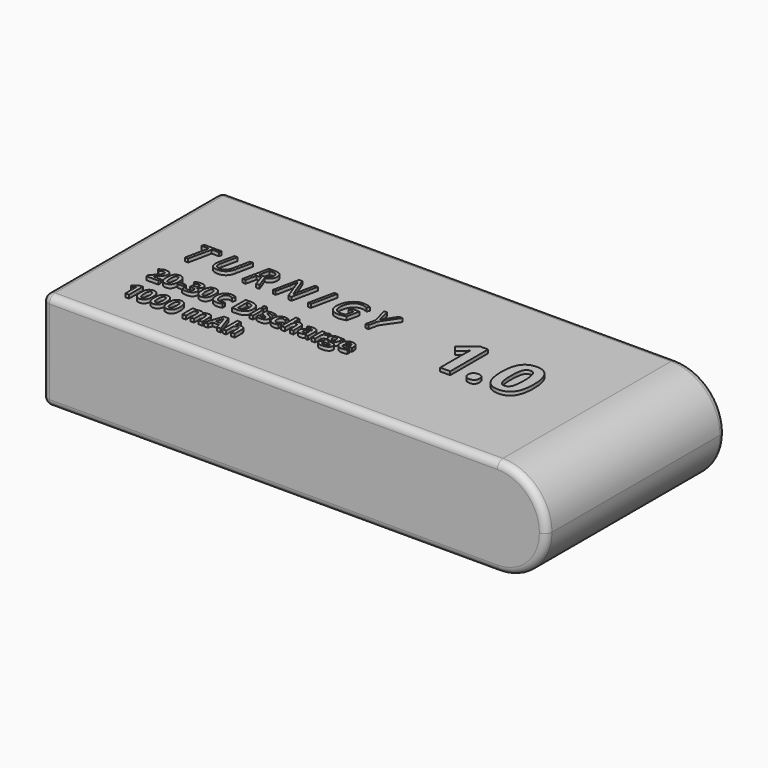
from build123d import *

# Parameters (mm, degrees)
F0_W           = 72
F0_H           = 14
F1_DEPTH       = 16
F2_R           = 6.99999
F3_R           = 1
F4_T1_DEPTH    = 30
F4_S5_W        = 1
F4_S5_H        = 1
F4_T6_DEPTH    = 1
F4_S11_W       = 1
F4_S11_H       = 1
F4_T12_DEPTH   = 1
F5_TEXT_SIZE   = 5.2058351343
F5_TEXT_SIZE_2 = 3.4440284883
F5_TEXT_SIZE_3 = 9.4785367967
F6_DEPTH       = 0.5


# Not quite as in the source:
# - a fillet or chamfer that OpenCascade refuses, or shapes differently, is made with other operations: its cross-section is extruded or revolved along the edge and cut away or added
# - a fillet or chamfer is up to 0.001 mm smaller than in the source, because OpenCascade refuses the exact size
# - Text() gives the source's letters only with a copy of the font that has no kerning and outlines rounded to 1/6400 em; it was checked with that copy


with BuildPart() as f1:
    # F0 (on Front) → F1 (new body, symmetric)
    with BuildSketch(Plane.XZ):
        Rectangle(F0_W, F0_H)
    extrude(amount=F1_DEPTH, both=True)

    # F2 (radius 7 in the source; OpenCascade refuses exactly that, so slightly less here)
    f2_edges = [f1.edges().sort_by_distance(p)[0] for p in [
        (36, 0, 7),
        (36, 0, -7),
    ]]
    fillet(f2_edges, radius=F2_R)

    # F3
    f3_edges = [f1.edges().sort_by_distance(p)[0] for p in [
        (-3.499995, -16, 7),
        (-3.499995, 16, 7),
        (-36, 0, -7),
        (-36, 16, 0),
        (-36, -16, 0),
    ]]
    fillet(f3_edges, radius=F3_R)

    # F4: fillet of radius 1 on 1 edges, made by hand

    # F4_s2 → F4_t1 (cut)
    with BuildSketch(Plane.XZ.offset(-15)):
        with BuildLine():
            ThreePointArc((-35, 7), (-35.7071067812, 6.7071067812), (-36, 6))
            Line((-36, 6), (-36, 7))
            Line((-36, 7), (-35, 7))
        make_face()
    extrude(amount=F4_T1_DEPTH, mode=Mode.SUBTRACT)


with BuildPart() as f4_tool4:
    # F4_s5 → F4_t6 (new body)
    with BuildSketch(Plane.XY.offset(6)):
        with Locations((-35.5, 15.5)):
            Rectangle(F4_S5_W, F4_S5_H)
    extrude(amount=F4_T6_DEPTH)

    # F4_s7 → F4_t8 (revolve, cut)
    with BuildSketch(Plane(origin=(-35, 15, 6), x_dir=(0.7071067812, -0.7071067812, 0), z_dir=(-0.7071067812, -0.7071067812, 0))):
        with BuildLine():
            ThreePointArc((0, -1), (1, 0), (0, 1))
            Line((0, 1), (0, -1))
        make_face()
    revolve(axis=Axis((-35, 15, 6), (0, 0, 1)), mode=Mode.SUBTRACT)


with BuildPart() as f1_1:
    add(f1.part)

    # F4_t3: cut F4_tool4
    add(f4_tool4.part, mode=Mode.SUBTRACT)


with BuildPart() as f4_tool10:
    # F4_s11 → F4_t12 (new body)
    with BuildSketch(Plane.XY.offset(6)):
        with Locations((-35.5, -15.5)):
            Rectangle(F4_S11_W, F4_S11_H)
    extrude(amount=F4_T12_DEPTH)

    # F4_s13 → F4_t14 (revolve, cut)
    with BuildSketch(Plane(origin=(-35, -15, 6), x_dir=(0.7071067812, 0.7071067812, 0), z_dir=(0.7071067812, -0.7071067812, 0))):
        with BuildLine():
            ThreePointArc((0, -1), (1, 0), (0, 1))
            Line((0, 1), (0, -1))
        make_face()
    revolve(axis=Axis((-35, -15, 6), (0, 0, 1)), mode=Mode.SUBTRACT)


with BuildPart() as f1_2:
    add(f1_1.part)

    # F4_t9: cut F4_tool10
    add(f4_tool10.part, mode=Mode.SUBTRACT)

    # F5 (on face) → F6 (join)
    with BuildSketch(Plane.XY.offset(7)):
        with Locations((-29.2242569853, 0)):
            Text('T U R N I G Y', F5_TEXT_SIZE, font='Open Sans', font_style=FontStyle.ITALIC, text_align=(TextAlign.LEFT, TextAlign.BOTTOM))
        with Locations((-29.1074220204, -6.2400386669)):
            Text('20-30C Discharge', F5_TEXT_SIZE_2, font='Open Sans', font_style=FontStyle.BOLD, text_align=(TextAlign.LEFT, TextAlign.BOTTOM))
        with Locations((-29.1074220204, -10.9239174109)):
            Text('1000 mAh', F5_TEXT_SIZE_2, font='Open Sans', font_style=FontStyle.BOLD, text_align=(TextAlign.LEFT, TextAlign.BOTTOM))
        with Locations((7.9452800564, -2.9998900136)):
            Text('1.0', F5_TEXT_SIZE_3, font='Open Sans', font_style=FontStyle.BOLD, text_align=(TextAlign.LEFT, TextAlign.BOTTOM))
    extrude(amount=F6_DEPTH)


solid = f1_2.part
